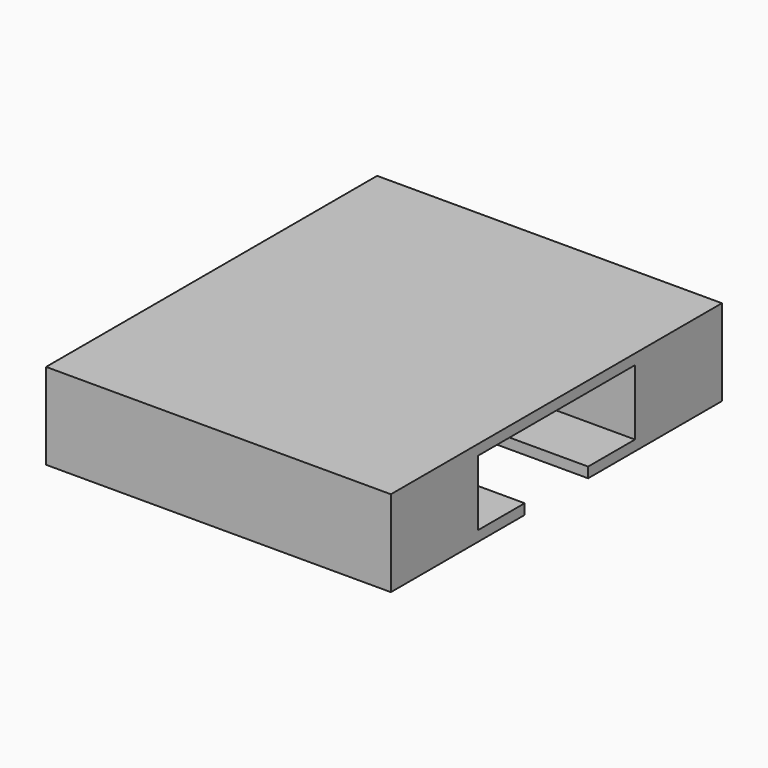
from build123d import *

# Parameters (mm, degrees)
F0_W     = 17
F0_H     = 3
F0_W_2   = 57
F0_W_3   = 28.5
F0_H_2   = 19
F1_DEPTH = 100


# Not quite as in the source:
# - a feature of the source that left no trace in its solid (it failed there, or was rolled back) is left out


with BuildPart() as f1:
    # F0 (on Right) → F1 (new body)
    with BuildSketch(Plane.YZ):
        with Locations((-31.5, 1.5)):
            Rectangle(F0_W, F0_H)
        Polygon((-68.5, 22), (-40, 22), (-40, 25), (-71.5, 25), (-71.5, 0), (-40, 0), (-40, 3), (-68.5, 3), align=None)
        with Locations((-11.5, 23.5)):
            Rectangle(F0_W_2, F0_H)
        Polygon((17, 3), (17, 0), (48.5, 0), (48.5, 25), (17, 25), (17, 22), (45.5, 22), (45.5, 3), align=None)
        with Locations((8.5, 1.5)):
            Rectangle(F0_W, F0_H)
        with Locations((31.25, 12.5)):
            Rectangle(F0_W_3, F0_H_2)
        with Locations((-54.25, 12.5)):
            Rectangle(F0_W_3, F0_H_2)
    extrude(amount=F1_DEPTH)


solid = f1.part
